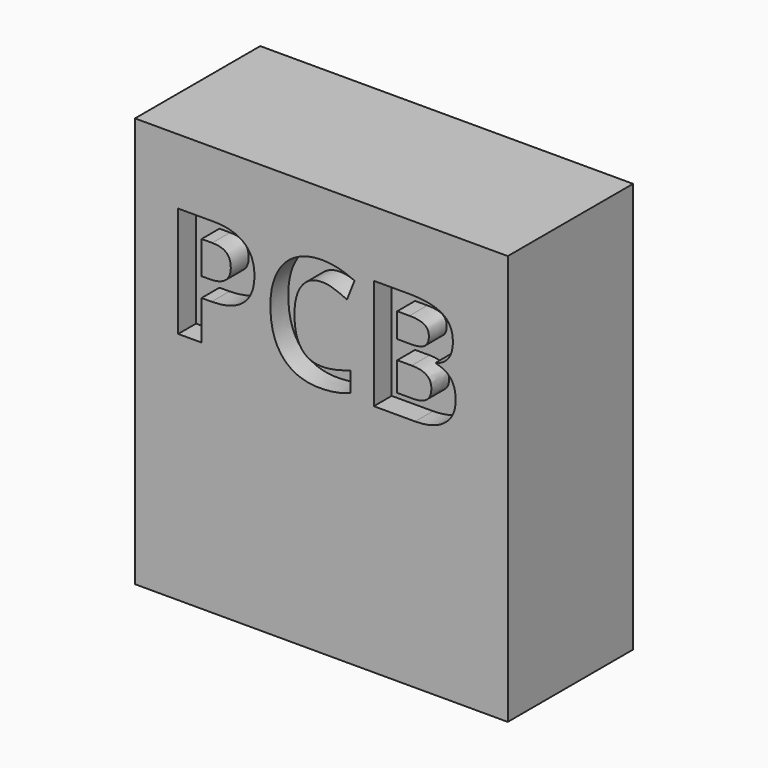
from build123d import *

# Parameters (mm, degrees)
F0_W         = 50
F0_H         = 55
F1_DEPTH     = 21
F3_TEXT_SIZE = 20.7406332872
F4_DEPTH     = 3


# Not quite as in the source:
# - Text() gives the source's letters only with a copy of the font that has no kerning and outlines rounded to 1/6400 em; it was checked with that copy


with BuildPart() as f1:
    # F0 (on Front) → F1 (new body)
    with BuildSketch(Plane.XZ):
        Rectangle(F0_W, F0_H)
    extrude(amount=F1_DEPTH)

    # F3 (on face) → F4 (cut)
    with BuildSketch(Plane.XZ.offset(21)):
        with Locations((-21.0699569434, 3.9335996844)):
            Text('PCB', F3_TEXT_SIZE, font='Open Sans', font_style=FontStyle.BOLD, text_align=(TextAlign.LEFT, TextAlign.BOTTOM))
    extrude(amount=-F4_DEPTH, mode=Mode.SUBTRACT)


solid = f1.part
